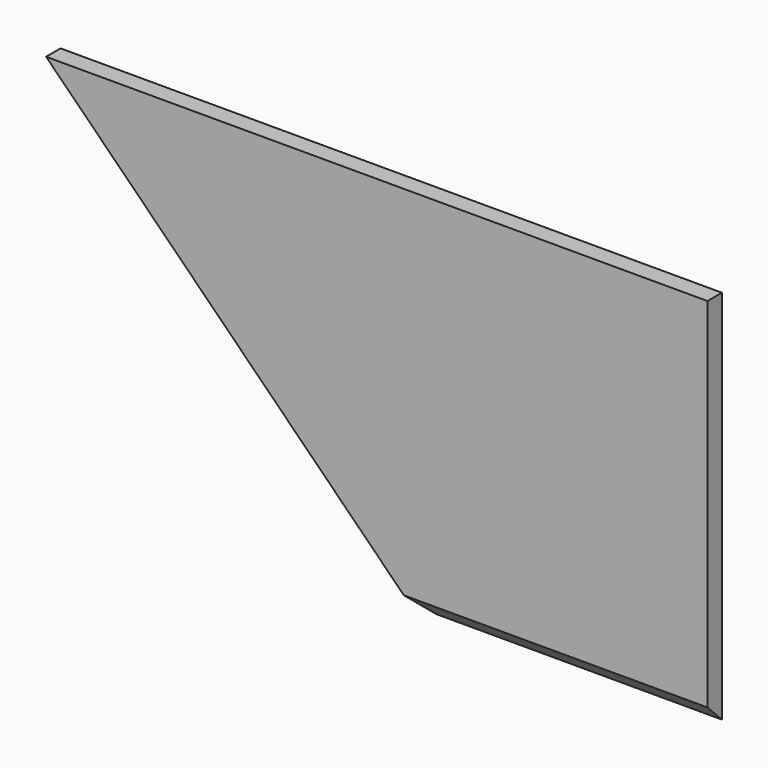
from build123d import *

# Parameters (mm, degrees)
F1_DEPTH = 15.875
F2_SIZE  = 15.87499


# Not quite as in the source:
# - a fillet or chamfer is up to 0.001 mm smaller than in the source, because OpenCascade refuses the exact size


with BuildPart() as f1:
    # F0 (on Front) → F1 (new body)
    with BuildSketch(Plane.XZ):
        Polygon((-250.825, 0), (0, 0), (0, 330.2), (-581.025, 330.2), align=None)
    extrude(amount=F1_DEPTH)

    # F2 (size 15.875 in the source; OpenCascade refuses exactly that, so slightly less here)
    f2_edges = [f1.edges().sort_by_distance(p)[0] for p in [
        (-125.4125, -15.875, 0),
    ]]
    chamfer(f2_edges, length=F2_SIZE)


solid = f1.part
